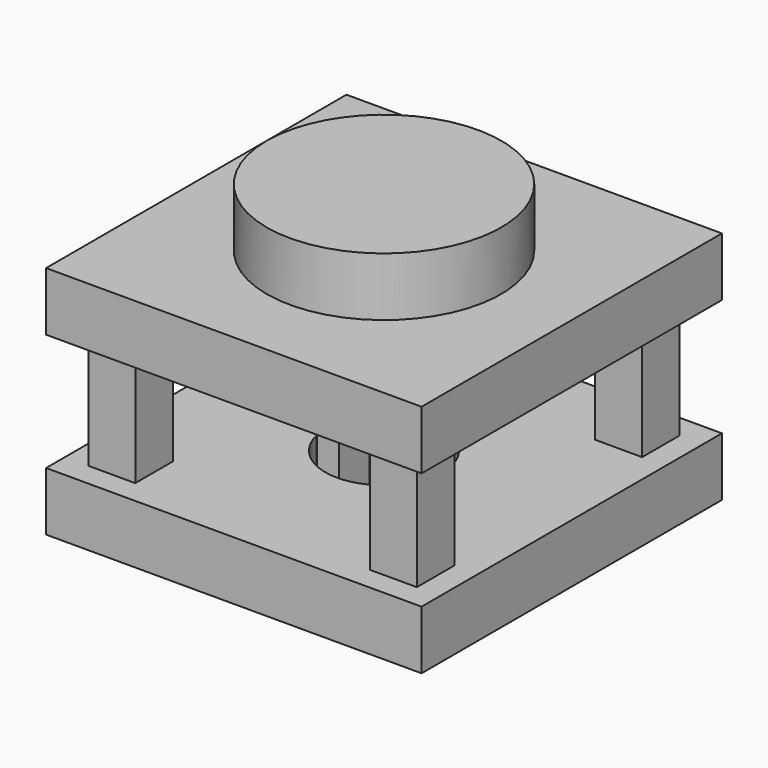
from build123d import *

# Parameters (mm, degrees)
F3_W      = 16
F3_H      = 16
F3_W_2    = 2
F3_H_2    = 2
F3_R      = 2.5
F4_DEPTH  = 2.5
F6_W      = 2
F6_H      = 2
F7_DEPTH  = 10
F11_DEPTH = 10
F12_SIZE2 = 2.5
F12_SIZE  = 0.25
F13_SIZE2 = 2.5
F13_SIZE  = 0.25
F14_SIZE2 = 2.5
F14_SIZE  = 0.25
F15_SIZE2 = 2.5
F15_SIZE  = 0.25


with BuildPart() as f4:
    # F3 (on offset) → F4 (new body)
    with BuildSketch(Plane.XY.offset(2.5)):
        Rectangle(F3_W, F3_H)
        with Locations((-6, -6)):
            Rectangle(F3_W_2, F3_H_2, mode=Mode.SUBTRACT)
        with Locations((6, -6)):
            Rectangle(F3_W_2, F3_H_2, mode=Mode.SUBTRACT)
        with Locations((-6, 6)):
            Rectangle(F3_W_2, F3_H_2, mode=Mode.SUBTRACT)
        Circle(F3_R, mode=Mode.SUBTRACT)
        with Locations((6, 6)):
            Rectangle(F3_W_2, F3_H_2, mode=Mode.SUBTRACT)
    extrude(amount=F4_DEPTH)


with BuildPart() as f5_1:
    # F5: copy of F4
    add(f4.part.moved(Location((0, 0, -7.5))))


with BuildPart() as f4_1:
    add(f4.part)

    # F6 (on face) → F7 (join)
    with BuildSketch(Plane.XY.offset(5)):
        with Locations((-6, -6)):
            Rectangle(F6_W, F6_H)
        with Locations((-6, 6)):
            Rectangle(F6_W, F6_H)
        with Locations((6, 6)):
            Rectangle(F6_W, F6_H)
        with Locations((6, -6)):
            Rectangle(F6_W, F6_H)
    extrude(amount=-F7_DEPTH)

    # F12
    f12_edges = [f4_1.edges().sort_by_distance(p)[0] for p in [
        (6, -7, -5),
        (7, -6, -5),
        (6, -5, -5),
        (5, -6, -5),
    ]]
    f12_side = f4_1.faces().sort_by_distance((6, -6, -5))[0]
    chamfer(f12_edges, length=F12_SIZE, length2=F12_SIZE2, reference=f12_side)

    # F13
    f13_edges = [f4_1.edges().sort_by_distance(p)[0] for p in [
        (6, 5, -5),
        (7, 6, -5),
        (6, 7, -5),
        (5, 6, -5),
    ]]
    f13_side = f4_1.faces().sort_by_distance((6, 6, -5))[0]
    chamfer(f13_edges, length=F13_SIZE, length2=F13_SIZE2, reference=f13_side)

    # F14
    f14_edges = [f4_1.edges().sort_by_distance(p)[0] for p in [
        (-6, 5, -5),
        (-5, 6, -5),
        (-6, 7, -5),
        (-7, 6, -5),
    ]]
    f14_side = f4_1.faces().sort_by_distance((-6, 6, -5))[0]
    chamfer(f14_edges, length=F14_SIZE, length2=F14_SIZE2, reference=f14_side)

    # F15
    f15_edges = [f4_1.edges().sort_by_distance(p)[0] for p in [
        (-6, -7, -5),
        (-5, -6, -5),
        (-6, -5, -5),
        (-7, -6, -5),
    ]]
    f15_side = f4_1.faces().sort_by_distance((-6, -6, -5))[0]
    chamfer(f15_edges, length=F15_SIZE, length2=F15_SIZE2, reference=f15_side)


with BuildPart() as f9:
    # F8 (on Front) → F9 (revolve)
    with BuildSketch(Plane.XZ):
        Polygon((0, -7.75), (0, 7.5), (-5, 7.5), (-5, 5), (-2.25, 5), (-2.25, -5.25), (-2.75, -5.25), (-2.25, -7.75), align=None)
    revolve(axis=Axis((0, 0, -0.0427132472), (0, 0, -1)))

    # F10 (on face) → F11 (cut)
    with BuildSketch(Plane(origin=(0, 0, -7.75), x_dir=(1, 0, 0), z_dir=(0, 0, -1))):
        with BuildLine():
            Line((1.5909902577, 1.5909902577), (2.2430448056, 1.5909902577))
            ThreePointArc((2.2430448056, 1.5909902577), (0, 2.75), (-2.2430448056, 1.5909902577))
            Line((-2.2430448056, 1.5909902577), (-1.5909902577, 1.5909902577))
            ThreePointArc((-1.5909902577, 1.5909902577), (0, 2.25), (1.5909902577, 1.5909902577))
        make_face()
        with BuildLine():
            Line((0.65, 1.5909902577), (1.5909902577, 1.5909902577))
            ThreePointArc((1.5909902577, 1.5909902577), (0, 2.25), (-1.5909902577, 1.5909902577))
            Line((-1.5909902577, 1.5909902577), (-0.65, 1.5909902577))
            Line((-0.65, 1.5909902577), (-0.65, -1.5909902577))
            Line((-0.65, -1.5909902577), (-1.5909902577, -1.5909902577))
            ThreePointArc((-1.5909902577, -1.5909902577), (0, -2.25), (1.5909902577, -1.5909902577))
            Line((1.5909902577, -1.5909902577), (0.65, -1.5909902577))
            Line((0.65, -1.5909902577), (0.65, 1.5909902577))
        make_face()
        with BuildLine():
            ThreePointArc((-2.2430448056, -1.5909902577), (0, -2.75), (2.2430448056, -1.5909902577))
            Line((2.2430448056, -1.5909902577), (1.5909902577, -1.5909902577))
            ThreePointArc((1.5909902577, -1.5909902577), (0, -2.25), (-1.5909902577, -1.5909902577))
            Line((-1.5909902577, -1.5909902577), (-2.2430448056, -1.5909902577))
        make_face()
    extrude(amount=-F11_DEPTH, mode=Mode.SUBTRACT)


solid = Compound([f5_1.part, f4_1.part, f9.part])
